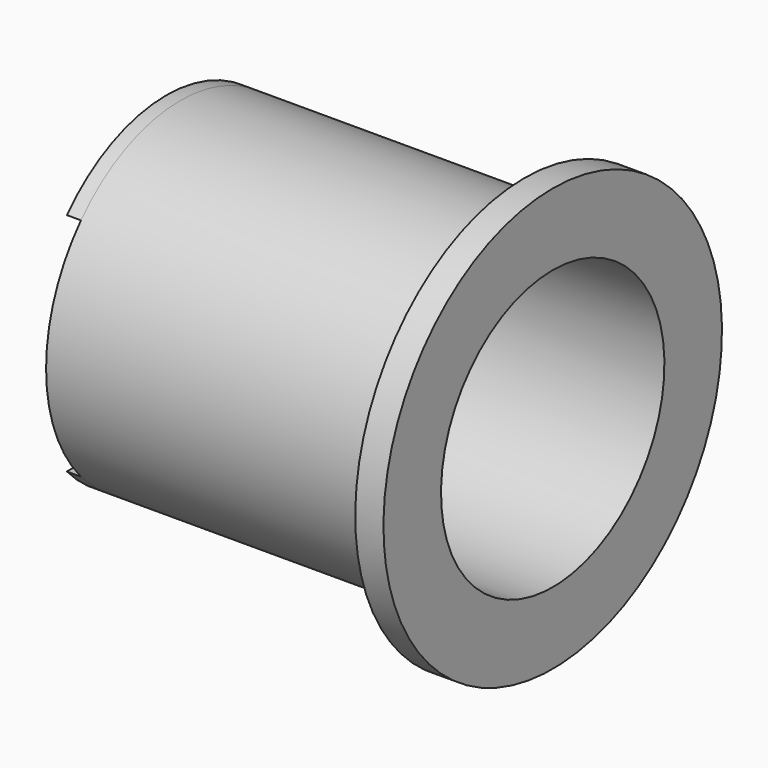
from build123d import *

# Parameters (mm, degrees)
F3_DEPTH = 0.5


# Not quite as in the source:
# - after a boolean that leaves OpenCascade's solid faulty, fix() repairs it


with BuildPart() as f1:
    # F0 (on Front) → F1 (revolve)
    with BuildSketch(Plane.XZ):
        Polygon((0, 5.95), (0, 2.5), (1, 2.5), (1, 4.95), (13.2, 4.95), (13.2, 7.5), (12.2, 7.5), (12.2, 5.95), align=None)
    revolve(axis=Axis((2.190093, 0, 0), (1, 0, 0)))

    # F2 (on face) → F3 (join)
    with BuildSketch(Plane(origin=(0, 0, 0), x_dir=(0, -1, 0), z_dir=(-1, 0, 0))):
        with BuildLine():
            ThreePointArc((4.404827, 4), (0, 5.95), (-4.404827, 4))
            Line((-4.404827, 4), (4.404827, 4))
        make_face()
        with BuildLine():
            Line((4.404827, -4), (-4.404827, -4))
            ThreePointArc((-4.404827, -4), (0, -5.95), (4.404827, -4))
        make_face()
    extrude(amount=F3_DEPTH)

    add(f1.part.fix(), mode=Mode.REPLACE)


solid = f1.part
